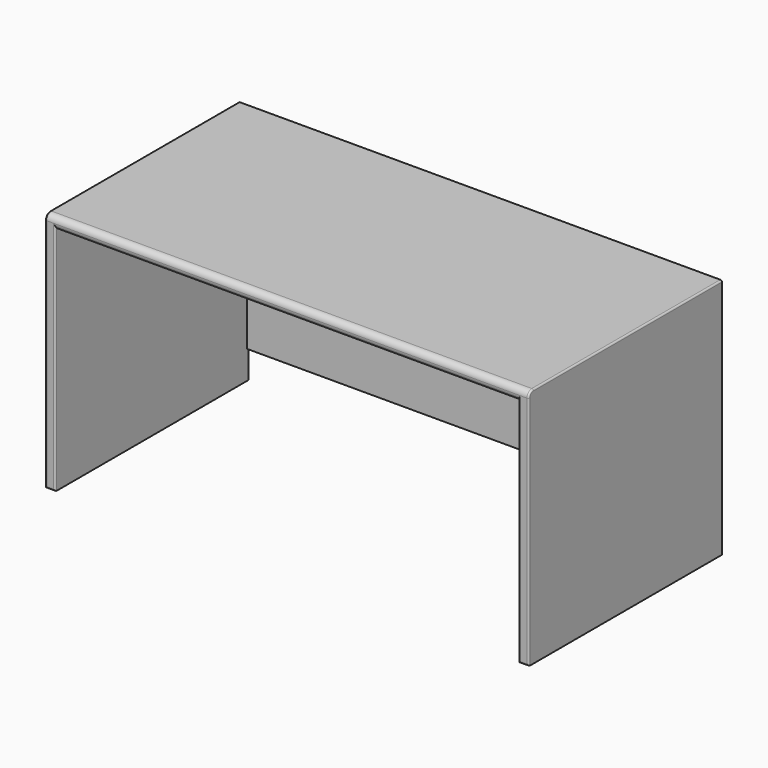
from build123d import *

# Parameters (mm, degrees)
F0_W     = 1460.5
F0_H     = 755.65
F0_H_2   = 6.35
F1_DEPTH = 38.1
F2_DEPTH = 723.9
F3_DEPTH = 635
F4_R     = 19.04999
F5_R     = 5.08


# Not quite as in the source:
# - a fillet or chamfer is up to 0.001 mm smaller than in the source, because OpenCascade refuses the exact size


with BuildPart() as f1:
    # F0 (on Top) → F1 (new body)
    with BuildSketch(Plane.XY):
        with Locations((762, 377.825)):
            Rectangle(F0_W, F0_H)
        Polygon((0, 762), (0, 0), (31.75, 0), (31.75, 755.65), (31.75, 762), align=None)
        with Locations((762, 758.825)):
            Rectangle(F0_W, F0_H_2)
        Polygon((1492.25, 755.65), (1492.25, 0), (1524, 0), (1524, 762), (1492.25, 762), align=None)
    extrude(amount=F1_DEPTH)

    # F0 (on Top) → F2 (join)
    with BuildSketch(Plane.XY):
        Polygon((0, 762), (0, 0), (31.75, 0), (31.75, 755.65), (31.75, 762), align=None)
        Polygon((1492.25, 755.65), (1492.25, 0), (1524, 0), (1524, 762), (1492.25, 762), align=None)
    extrude(amount=-F2_DEPTH)

    # F0 (on Top) → F3 (join)
    with BuildSketch(Plane.XY):
        with Locations((762, 758.825)):
            Rectangle(F0_W, F0_H_2)
    extrude(amount=-F3_DEPTH)

    # F4 (radius 19.05 in the source; OpenCascade refuses exactly that, so slightly less here)
    f4_edges = [f1.edges().sort_by_distance(p)[0] for p in [
        (762, 0, 38.1),
        (762, 0, 0),
    ]]
    fillet(f4_edges, radius=F4_R)

    # F5
    f5_edges = [f1.edges().sort_by_distance(p)[0] for p in [
        (1524, 0, -352.424995),
        (762, 0, 19.05001),
        (1508.125, 0, -723.9),
        (0, 0, -352.424995),
        (1492.25, 0, -361.95),
        (15.875, 0, -723.9),
        (1492.25, 0, 9.524995),
        (31.75, 0, -361.95),
        (762, 0, 19.04999),
        (31.75, 0, 9.524995),
    ]]
    fillet(f5_edges, radius=F5_R)


solid = f1.part
